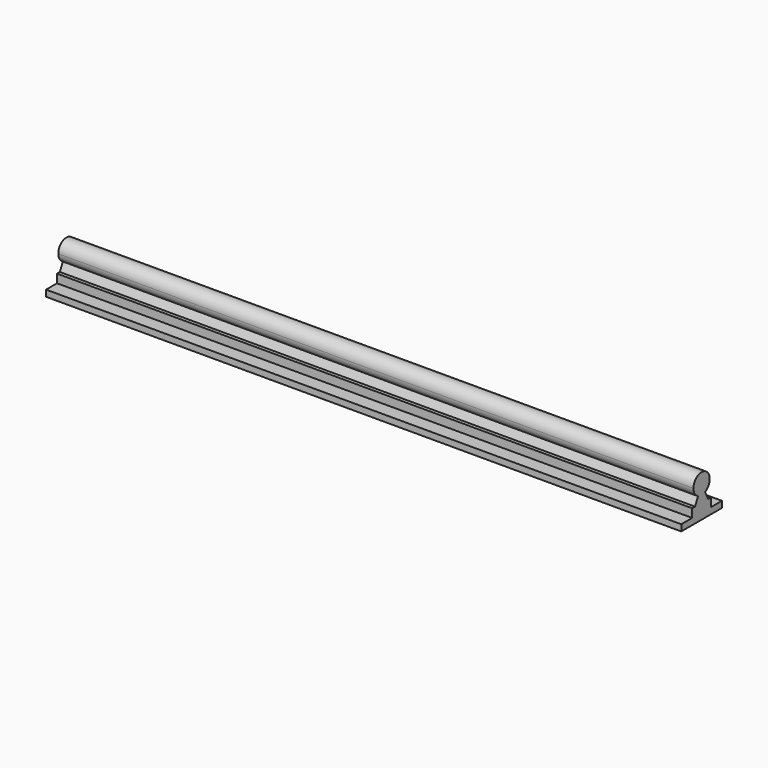
from build123d import *

# Parameters (mm, degrees)
F0_W     = 500
F0_H     = 40
F1_DEPTH = 5
F3_DEPTH = 500
F5_DEPTH = 500


with BuildPart() as f1:
    # F0 (on Top) → F1 (new body)
    with BuildSketch(Plane.XY):
        Rectangle(F0_W, F0_H)
    extrude(amount=F1_DEPTH)

    # F2 (on face) → F3 (join, through all)
    with BuildSketch(Plane.YZ.offset(250)):
        Polygon((-9.25, 11.7), (-9.25, 0), (9.25, 0), (9.25, 11.7), (6.4414839943, 11.7), (-6.4414839943, 11.7), align=None)
        with BuildLine():
            Line((-6.3045076751, 11.9828207053), (-6.4414839943, 11.7))
            Line((-6.4414839943, 11.7), (6.4414839943, 11.7))
            Line((6.4414839943, 11.7), (5.346455176, 13.9609515597))
            Line((5.346455176, 13.9609515597), (3.4871191548, 17.8))
            ThreePointArc((3.4871191548, 17.8), (0, 17), (-3.4871191548, 17.8))
            Line((-3.4871191548, 17.8), (-6.3045076751, 11.9828207053))
        make_face()
    extrude(amount=-F3_DEPTH)

    # F4 (on face) → F5 (join, through all)
    with BuildSketch(Plane(origin=(-250, 0, 0), x_dir=(0, -1, 0), z_dir=(-1, 0, 0))):
        with BuildLine():
            ThreePointArc((3.4871191548, 17.8), (6.7785305649, 20.7512915632), (8, 25))
            ThreePointArc((8, 25), (-4.2487084368, 31.7785305649), (-3.4871191548, 17.8))
            ThreePointArc((-3.4871191548, 17.8), (0, 17), (3.4871191548, 17.8))
        make_face()
    extrude(amount=-F5_DEPTH)


solid = f1.part
